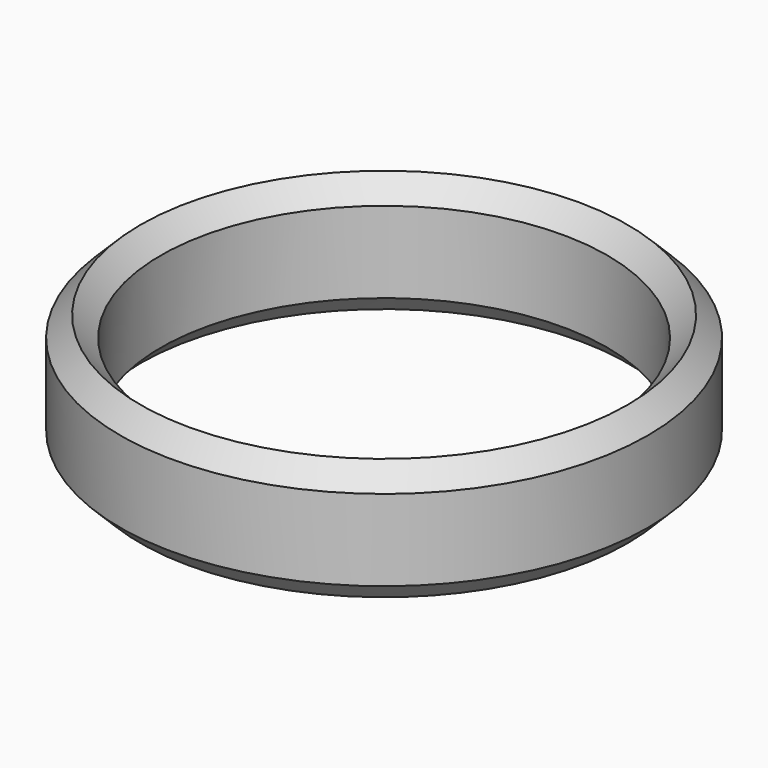
from build123d import *

# Parameters (mm, degrees)
F0_R     = 49.53
F0_R_2   = 41.91
F1_DEPTH = 25.4
F2_SIZE  = 5.08
F4_SIZE  = 5.08


# Not quite as in the source:
# - a fillet or chamfer that OpenCascade refuses, or shapes differently, is made with other operations: its cross-section is extruded or revolved along the edge and cut away or added


with BuildPart() as f1:
    # F0 (on Top) → F1 (new body)
    with BuildSketch(Plane.XY):
        Circle(F0_R)
        Circle(F0_R_2, mode=Mode.SUBTRACT)
    extrude(amount=F1_DEPTH)

    # F2
    f2_edges = [f1.edges().sort_by_distance(p)[0] for p in [
        (-41.91, 0, 25.4),
    ]]
    chamfer(f2_edges, length=F2_SIZE)

    # F3: chamfer of 5.08 on 1 edges, made by hand

    # F3_s1 → F3_t2 (revolve, cut)
    with BuildSketch(Plane.XZ):
        Polygon((44.45, 25.4), (49.53, 20.32), (49.53, 25.4), align=None)
    revolve(axis=Axis((0, 0, 25.4), (0, 0, 1)), mode=Mode.SUBTRACT)

    # F4
    f4_edges = [f1.edges().sort_by_distance(p)[0] for p in [
        (-49.53, 0, 0),
    ]]
    chamfer(f4_edges, length=F4_SIZE)

    # F5: chamfer of 5.08 on 1 edges, made by hand

    # F5_s1 → F5_t2 (revolve, cut)
    with BuildSketch(Plane.XZ):
        Polygon((46.99, 0), (41.91, 5.08), (41.91, 0), align=None)
    revolve(axis=Axis((0, 0, 0), (0, 0, 1)), mode=Mode.SUBTRACT)


solid = f1.part
